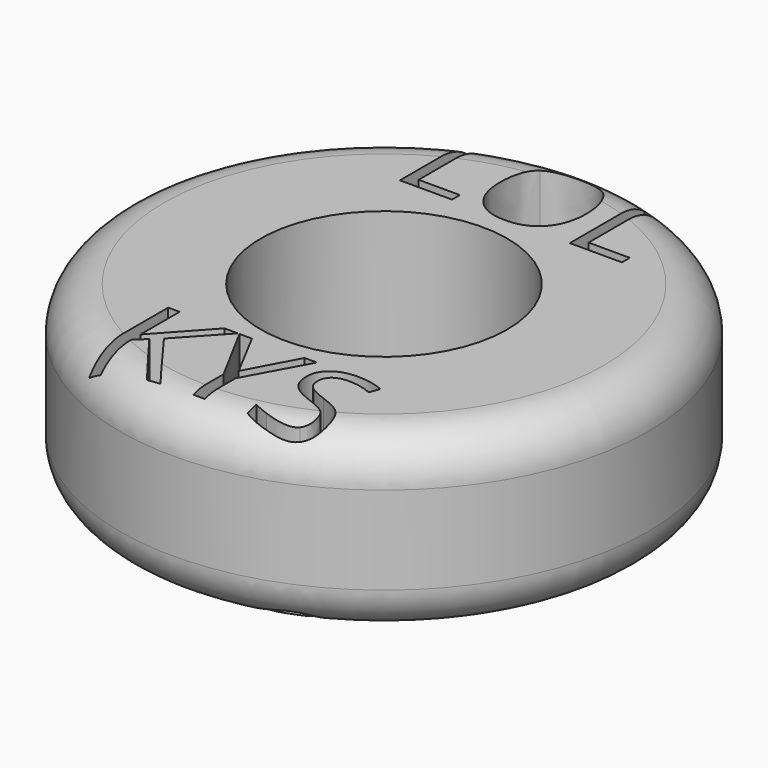
from build123d import *

# Parameters (mm, degrees)
F0_R     = 30
F0_R_2   = 14
F1_DEPTH = 20


# Not quite as in the source:
# - a fillet or chamfer that OpenCascade refuses, or shapes differently, is made with other operations: its cross-section is extruded or revolved along the edge and cut away or added


with BuildPart() as f1:
    # F0 (on Top) → F1 (new body)
    with BuildSketch(Plane.XY):
        Circle(F0_R)
        Polygon((-8.6969163566, -20.3703688444), (-4.0202842292, -26.7105668598), (-5.5538073559, -26.7105668598), (-9.6391129657, -21.2733072615), (-10.8144050901, -22.3161029877), (-10.8144050901, -26.7105668598), (-12.1172863386, -26.7105668598), (-12.1172863386, -15.4998993938), (-10.8144050901, -15.4998993938), (-10.8144050901, -21.0598408422), (-5.7304692202, -15.4998993938), (-4.1895851824, -15.4998993938), align=None, mode=Mode.SUBTRACT)
        Polygon((-2.5947211305, -15.4998993938), (0.3741796429, -21.1064599453), (3.3627095124, -15.4998993938), (4.773550789, -15.4998993938), (1.0317543597, -22.3627220907), (1.0317543597, -26.7105668598), (-0.2858487108, -26.7105668598), (-0.2858487108, -22.4240630158), (-4.0202842292, -15.4998993938), align=None, mode=Mode.SUBTRACT)
        with BuildLine():
            add(Edge.make_bspline(
                [(11.9774290294, -21.8572728681), (12.6399110202, -22.578642147), (12.6399110202, -23.7269442643)],
                knots=[0, 0, 0, 1, 1, 1], degree=2))
            add(Edge.make_bspline(
                [(12.6399110202, -23.7269442643), (12.6399110202, -25.206487377), (11.5664448314, -26.035816684)],
                knots=[0, 0, 0, 1, 1, 1], degree=2))
            add(Edge.make_bspline(
                [(11.5664448314, -26.035816684), (10.4929786427, -26.865145991), (8.6527508905, -26.865145991)],
                knots=[0, 0, 0, 1, 1, 1], degree=2))
            add(Edge.make_bspline(
                [(8.6527508905, -26.865145991), (6.6603976442, -26.865145991), (5.585704637, -26.3498822204)],
                knots=[0, 0, 0, 1, 1, 1], degree=2))
            Line((5.585704637, -26.3498822204), (5.585704637, -25.0936200749))
            add(Edge.make_bspline(
                [(5.585704637, -25.0936200749), (6.2776302718, -25.3831492412), (7.0897841197, -25.5524501944)],
                knots=[0, 0, 0, 1, 1, 1], degree=2))
            add(Edge.make_bspline(
                [(7.0897841197, -25.5524501944), (7.9019379677, -25.7217511476), (8.6993699936, -25.7217511476)],
                knots=[0, 0, 0, 1, 1, 1], degree=2))
            add(Edge.make_bspline(
                [(8.6993699936, -25.7217511476), (10.0022512421, -25.7217511476), (10.6622795959, -25.2273432916)],
                knots=[0, 0, 0, 1, 1, 1], degree=2))
            add(Edge.make_bspline(
                [(10.6622795959, -25.2273432916), (11.3223079496, -24.7329354355), (11.3223079496, -23.8496261145)],
                knots=[0, 0, 0, 1, 1, 1], degree=2))
            add(Edge.make_bspline(
                [(11.3223079496, -23.8496261145), (11.3223079496, -23.2681141448), (11.0879856159, -22.8963881388)],
                knots=[0, 0, 0, 1, 1, 1], degree=2))
            add(Edge.make_bspline(
                [(11.0879856159, -22.8963881388), (10.8536632821, -22.5246621329), (10.305275412, -22.2093697781)],
                knots=[0, 0, 0, 1, 1, 1], degree=2))
            add(Edge.make_bspline(
                [(10.305275412, -22.2093697781), (9.7568875418, -21.8940774232), (8.6380290685, -21.4965882287)],
                knots=[0, 0, 0, 1, 1, 1], degree=2))
            add(Edge.make_bspline(
                [(8.6380290685, -21.4965882287), (7.0750622977, -20.9371589921), (6.4039925774, -20.1703974287)],
                knots=[0, 0, 0, 1, 1, 1], degree=2))
            add(Edge.make_bspline(
                [(6.4039925774, -20.1703974287), (5.7329228572, -19.4036358653), (5.7329228572, -18.1694564529)],
                knots=[0, 0, 0, 1, 1, 1], degree=2))
            add(Edge.make_bspline(
                [(5.7329228572, -18.1694564529), (5.7329228572, -16.8739361154), (6.7057899288, -16.107174552)],
                knots=[0, 0, 0, 1, 1, 1], degree=2))
            add(Edge.make_bspline(
                [(6.7057899288, -16.107174552), (7.6786570004, -15.3404129886), (9.2833356003, -15.3404129886)],
                knots=[0, 0, 0, 1, 1, 1], degree=2))
            add(Edge.make_bspline(
                [(9.2833356003, -15.3404129886), (10.9542623992, -15.3404129886), (12.3577427648, -15.9538222393)],
                knots=[0, 0, 0, 1, 1, 1], degree=2))
            Line((12.3577427648, -15.9538222393), (11.9504390224, -17.0874025346))
            add(Edge.make_bspline(
                [(11.9504390224, -17.0874025346), (10.5616804788, -16.5058905649), (9.2514383192, -16.5058905649)],
                knots=[0, 0, 0, 1, 1, 1], degree=2))
            add(Edge.make_bspline(
                [(9.2514383192, -16.5058905649), (8.216003504, -16.5058905649), (7.6332647159, -16.9499988624)],
                knots=[0, 0, 0, 1, 1, 1], degree=2))
            add(Edge.make_bspline(
                [(7.6332647159, -16.9499988624), (7.0505259277, -17.39410716), (7.0505259277, -18.1841782749)],
                knots=[0, 0, 0, 1, 1, 1], degree=2))
            add(Edge.make_bspline(
                [(7.0505259277, -18.1841782749), (7.0505259277, -18.7656902446), (7.2652191654, -19.138643069)],
                knots=[0, 0, 0, 1, 1, 1], degree=2))
            add(Edge.make_bspline(
                [(7.2652191654, -19.138643069), (7.4799124032, -19.5115958934), (7.9902688998, -19.8219809743)],
                knots=[0, 0, 0, 1, 1, 1], degree=2))
            add(Edge.make_bspline(
                [(7.9902688998, -19.8219809743), (8.5006253964, -20.1323660551), (9.5507820336, -20.5077725166)],
                knots=[0, 0, 0, 1, 1, 1], degree=2))
            add(Edge.make_bspline(
                [(9.5507820336, -20.5077725166), (11.3149470386, -21.1359035893), (11.9774290294, -21.8572728681)],
                knots=[0, 0, 0, 1, 1, 1], degree=2))
        make_face(mode=Mode.SUBTRACT)
        Polygon((-5.4187737125, 16.4271035947), (-11.3369023302, 16.4271035947), (-11.3369023302, 27.0434874402), (-10.1030875301, 27.0434874402), (-10.1030875301, 17.5447399768), (-5.4187737125, 17.5447399768), align=None, mode=Mode.SUBTRACT)
        Circle(F0_R_2, mode=Mode.SUBTRACT)
        with BuildLine():
            add(Edge.make_bspline(
                [(4.3123305871, 25.758554136), (5.5972638912, 24.3063239099), (5.5972638912, 21.7503987118)],
                knots=[0, 0, 0, 1, 1, 1], degree=2))
            add(Edge.make_bspline(
                [(5.5972638912, 21.7503987118), (5.5972638912, 19.2014442188), (4.3076834504, 17.7410815033)],
                knots=[0, 0, 0, 1, 1, 1], degree=2))
            add(Edge.make_bspline(
                [(4.3076834504, 17.7410815033), (3.0181030095, 16.2807187879), (0.7247410363, 16.2807187879)],
                knots=[0, 0, 0, 1, 1, 1], degree=2))
            add(Edge.make_bspline(
                [(0.7247410363, 16.2807187879), (-1.6197394408, 16.2807187879), (-2.8942166873, 17.7155222514)],
                knots=[0, 0, 0, 1, 1, 1], degree=2))
            add(Edge.make_bspline(
                [(-2.8942166873, 17.7155222514), (-4.1686939338, 19.1503257148), (-4.1686939338, 21.764340122)],
                knots=[0, 0, 0, 1, 1, 1], degree=2))
            add(Edge.make_bspline(
                [(-4.1686939338, 21.764340122), (-4.1686939338, 24.3574424138), (-2.8907313348, 25.784113388)],
                knots=[0, 0, 0, 1, 1, 1], degree=2))
            add(Edge.make_bspline(
                [(-2.8907313348, 25.784113388), (-1.6127687357, 27.2107843622), (0.7386824465, 27.2107843622)],
                knots=[0, 0, 0, 1, 1, 1], degree=2))
            add(Edge.make_bspline(
                [(0.7386824465, 27.2107843622), (3.027397283, 27.2107843622), (4.3123305871, 25.758554136)],
                knots=[0, 0, 0, 1, 1, 1], degree=2))
        make_face(mode=Mode.SUBTRACT)
        Polygon((13.8807851014, 16.4271035947), (7.9626564836, 16.4271035947), (7.9626564836, 27.0434874402), (9.1964712838, 27.0434874402), (9.1964712838, 17.5447399768), (13.8807851014, 17.5447399768), align=None, mode=Mode.SUBTRACT)
    extrude(amount=F1_DEPTH)

    # F2: fillet of radius 5 on 3 edges, made by hand

    # F2_s1 → F2_t2 (revolve, cut)
    with BuildSketch(Plane.XZ):
        with BuildLine():
            ThreePointArc((30, 5), (28.5355339059, 1.4644660941), (25, 0))
            Line((25, 0), (30, 0))
            Line((30, 0), (30, 5))
        make_face()
    revolve(axis=Axis((0, 0, 0), (0, 0, 1)), mode=Mode.SUBTRACT)

    # F2_s3 → F2_t4 (revolve, cut)
    with BuildSketch(Plane.XZ):
        with BuildLine():
            ThreePointArc((30, 15), (28.5355339059, 18.5355339059), (25, 20))
            Line((25, 20), (30, 20))
            Line((30, 20), (30, 15))
        make_face()
    revolve(axis=Axis((0, 0, 20), (0, 0, 1)), mode=Mode.SUBTRACT)


solid = f1.part
